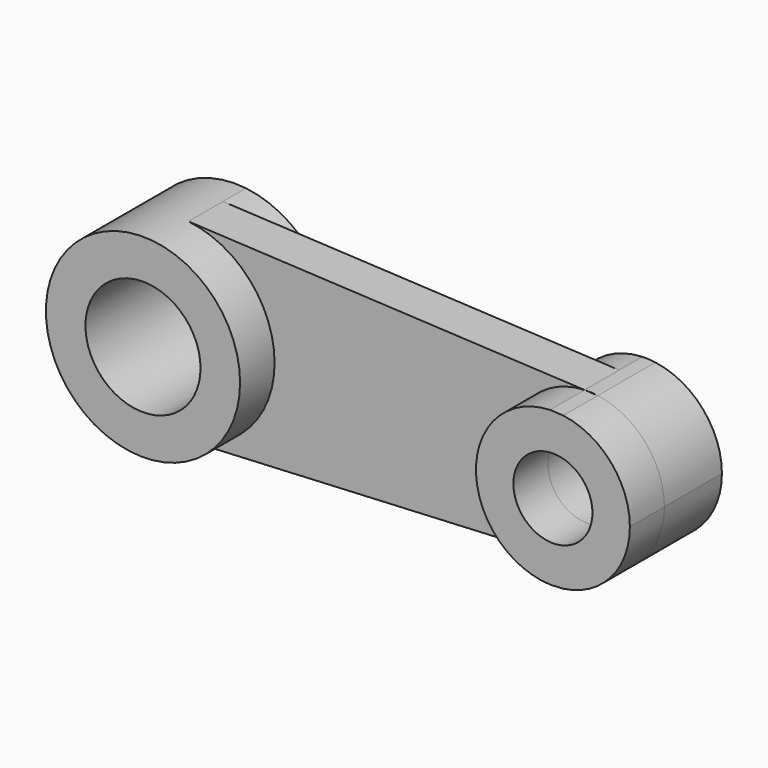
from build123d import *
from build123d import SkipClean  # not in build123d's __all__

# Parameters (mm, degrees)
F0_R     = 17.4625
F1_DEPTH = 31.75
F2_DEPTH = 31.75
F0_R_2   = 25.4
F3_DEPTH = 50.8
F4_DEPTH = 12.7
F5_DEPTH = 50.8


with BuildPart() as f1:
    # F0 (on Front) → F1 (new body)
    with BuildSketch(Plane.XZ):
        with BuildLine():
            ThreePointArc((137.8952277792, 72.3404701197), (134.9898494581, 72.609247784), (132.0721238048, 72.6277311095))
            Line((132.0721238048, 72.6277311095), (137.8952277792, 72.3404701197))
        make_face()
        with BuildLine():
            Line((137.8952277792, 5.0155493856), (132.0808217973, 4.7279708331))
            ThreePointArc((132.0808217973, 4.7279708331), (134.9941960526, 4.7469864233), (137.8952277792, 5.0155493856))
        make_face()
        with BuildLine():
            Line((137.8952277792, 72.3404701197), (132.0721238048, 72.6277311095))
            ThreePointArc((132.0721238048, 72.6277311095), (99.3434793984, 38.6736578588), (132.0808217973, 4.7279708331))
            Line((132.0808217973, 4.7279708331), (137.8952277792, 5.0155493856))
            ThreePointArc((137.8952277792, 5.0155493856), (158.9060092226, 16.333410504), (167.2884791197, 38.6780097526))
            ThreePointArc((167.2884791197, 38.6780097526), (158.9060092226, 61.0226090013), (137.8952277792, 72.3404701197))
        make_face()
        with Locations((133.3159791197, 38.6780097526)):
            Circle(F0_R, mode=Mode.SUBTRACT)
    extrude(amount=F1_DEPTH)

    # F0 (on Front) → F2 (join)
    with BuildSketch(Plane.XZ):
        with BuildLine():
            ThreePointArc((-42.8278144375, 81.2557634421), (-15.6881628684, 67.2156297522), (-4.7965205083, 38.6664061547))
            ThreePointArc((-4.7965205083, 38.6664061547), (-15.6881628684, 10.1171825573), (-42.8278144375, -3.9229511326))
            Line((-42.8278144375, -3.9229511326), (132.0808217973, 4.7279708331))
            ThreePointArc((132.0808217973, 4.7279708331), (99.3434793984, 38.6736578588), (132.0721238048, 72.6277311095))
            Line((132.0721238048, 72.6277311095), (-42.8278144375, 81.2557634421))
        make_face()
    extrude(amount=F2_DEPTH)

    # F0 (on Front) → F3 (join)
    with BuildSketch(Plane.XZ):
        with BuildLine():
            ThreePointArc((-42.8278144375, -3.9229511326), (-15.6881628684, 10.1171825573), (-4.7965205083, 38.6664061547))
            ThreePointArc((-4.7965205083, 38.6664061547), (-15.6881628684, 67.2156297522), (-42.8278144375, 81.2557634421))
            ThreePointArc((-42.8278144375, 81.2557634421), (-90.5215205083, 38.6664061547), (-42.8278144375, -3.9229511326))
        make_face()
        with Locations((-47.6590205083, 38.6664061547)):
            Circle(F0_R_2, mode=Mode.SUBTRACT)
    extrude(amount=F3_DEPTH)

    # F0 (on Front) → F4 (cut)
    with BuildSketch(Plane.XZ):
        with BuildLine():
            ThreePointArc((-42.8278144375, 81.2557634421), (-15.6881628684, 67.2156297522), (-4.7965205083, 38.6664061547))
            ThreePointArc((-4.7965205083, 38.6664061547), (-15.6881628684, 10.1171825573), (-42.8278144375, -3.9229511326))
            Line((-42.8278144375, -3.9229511326), (132.0808217973, 4.7279708331))
            ThreePointArc((132.0808217973, 4.7279708331), (99.3434793984, 38.6736578588), (132.0721238048, 72.6277311095))
            Line((132.0721238048, 72.6277311095), (-42.8278144375, 81.2557634421))
        make_face()
    with SkipClean():  # cleaning this boolean's faces spoils the solid; the shape is the same uncleaned
        extrude(amount=F4_DEPTH, mode=Mode.SUBTRACT)

    # F0 (on Front) → F5 (join)
    with BuildSketch(Plane.XZ):
        with BuildLine():
            Line((137.8952277792, 72.3404701197), (132.0721238048, 72.6277311095))
            ThreePointArc((132.0721238048, 72.6277311095), (99.3434793984, 38.6736578588), (132.0808217973, 4.7279708331))
            Line((132.0808217973, 4.7279708331), (137.8952277792, 5.0155493856))
            ThreePointArc((137.8952277792, 5.0155493856), (158.9060092226, 16.333410504), (167.2884791197, 38.6780097526))
            ThreePointArc((167.2884791197, 38.6780097526), (158.9060092226, 61.0226090013), (137.8952277792, 72.3404701197))
        make_face()
        with Locations((133.3159791197, 38.6780097526)):
            Circle(F0_R, mode=Mode.SUBTRACT)
    with SkipClean():  # cleaning this boolean's faces spoils the solid; the shape is the same uncleaned
        extrude(amount=F5_DEPTH)


solid = f1.part
